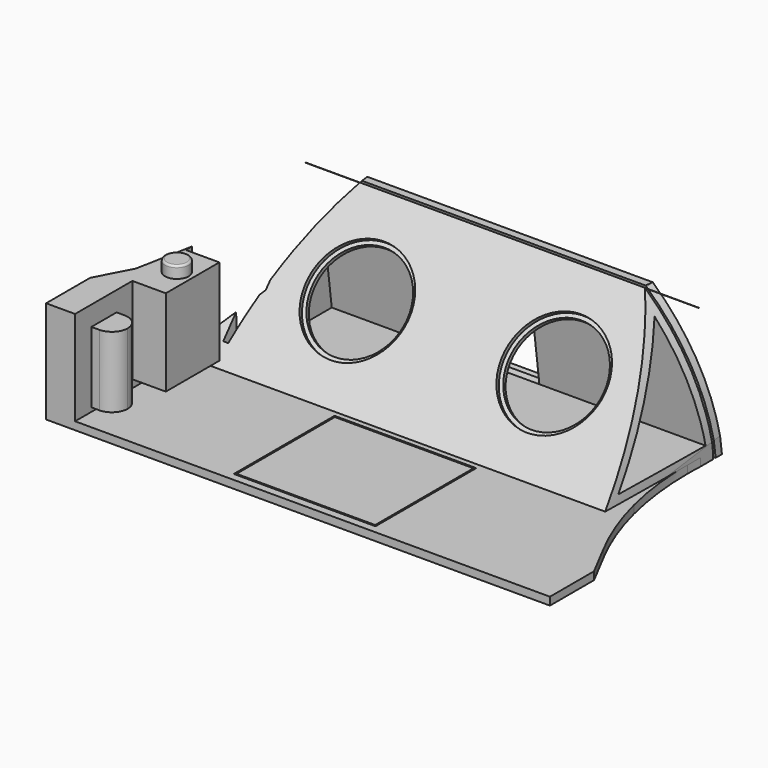
from build123d import *

# Parameters (mm, degrees)
F1_DEPTH  = 25.4
F3_DEPTH  = 1270
F5_W      = 457.2
F5_H      = 406.4
F6_DEPTH  = 25.4
F7_W      = 447.04
F7_H      = 396.24
F8_DEPTH  = 25.4
F10_DEPTH = 1358.9
F11_R     = 165.1
F12_DEPTH = 12.7
F14_DEPTH = 1206.5
F16_DEPTH = 25.4
F17_R     = 152.4
F18_DEPTH = 25.4
F4_W      = 203.2
F4_H      = 397.8725210062
F19_DEPTH = 25.4
F21_DEPTH = 25.4
F23_DEPTH = 459.74
F24_W     = 185.8009562355
F24_H     = 25.4
F25_DEPTH = 127
F27_DEPTH = 25.4
F29_DEPTH = 25.4
F31_DEPTH = 304.8
F32_W     = 215.9
F32_H     = 279.4
F33_DEPTH = 107.95
F34_W     = 101.6
F34_H     = 228.6
F35_DEPTH = 76.2
F36_R     = 50.8
F37_R     = 50.79999
F38_R     = 38.1
F39_DEPTH = 38.1
F40_R     = 6.35
F42_DEPTH = 508
F44_DEPTH = 406.4


# Not quite as in the source:
# - a fillet or chamfer is up to 0.001 mm smaller than in the source, because OpenCascade refuses the exact size


with BuildPart() as f1:
    # F0 (on Top) → F1 (new body)
    with BuildSketch(Plane.XY):
        Polygon((633.9916200739, 381), (-636.0083799261, 381), (-636.0083799261, 279.4), (-585.2083799261, 279.4), (-585.2083799261, 101.6), (-720.2711577423, -25.9932654437), (-755.401483878, -208.8168415053), (-813.8083799261, -320.4935488224), (-813.8083799261, -498.2935488224), (-636.0083799261, -498.2935488224), (633.9916200739, -498.2935488224), (811.7916200739, -498.2935488224), (811.7916200739, -320.4935488224), (753.3847240259, -208.8168415053), (718.2543978901, -25.9932654437), (583.1916200739, 101.6), (583.1916200739, 279.4), (633.9916200739, 279.4), align=None)
    extrude(amount=F1_DEPTH)

    # F5 (on face) → F6 (cut)
    with BuildSketch(Plane.XY.offset(25.4)):
        with Locations((0, -269.6935488224)):
            Rectangle(F5_W, F5_H)
    extrude(amount=-F6_DEPTH, mode=Mode.SUBTRACT)


with BuildPart() as f3:
    # F2 (on face) → F3 (new body)
    with BuildSketch(Plane.YZ.offset(633.9916200739)):
        Polygon((355.6, 457.2), (330.2, 457.2), (392.1093138361, 0), (417.5093138361, 0), align=None)
    extrude(amount=-F3_DEPTH)

    # F4 (on face) → F19 (cut)
    with BuildSketch(Plane(origin=(0, 385.0491351938, 52.1393870364), x_dir=(1, 0, 0), z_dir=(0, -0.9909562863, -0.1341850913))):
        with Locations((0, 184.4210364421)):
            Rectangle(F4_W, F4_H)
    extrude(amount=-F19_DEPTH, mode=Mode.SUBTRACT)

    # F20 (on face) → F21 (cut)
    with BuildSketch(Plane(origin=(0, 385.0491351938, 52.1393870364), x_dir=(1, 0, 0), z_dir=(0, -0.9909562863, -0.1341850913))):
        with BuildLine():
            ThreePointArc((-636.0083799261, -52.615224061), (-589.7862100298, 194.7614898935), (-457.3568999767, 408.7572969452))
            Line((-457.3568999767, 408.7572969452), (-636.0083799261, 408.7572969452))
            Line((-636.0083799261, 408.7572969452), (-636.0083799261, -52.615224061))
        make_face()
        with BuildLine():
            Line((633.9916200739, 408.7572969452), (457.3568999767, 408.7572969452))
            ThreePointArc((457.3568999767, 408.7572969452), (579.8251172789, 219.089488202), (633.9916200739, -0.0869975296))
            Line((633.9916200739, -0.0869975296), (633.9916200739, 408.7572969452))
        make_face()
    extrude(amount=-F21_DEPTH, mode=Mode.SUBTRACT)


with BuildPart() as f8:
    # F7 (on face) → F8 (new body)
    with BuildSketch(Plane.XY.offset(25.4)):
        with Locations((0, -269.6935488224)):
            Rectangle(F7_W, F7_H)
    extrude(amount=-F8_DEPTH)


with BuildPart() as f10:
    # F9 (on face) → F10 (new body)
    with BuildSketch(Plane.YZ.offset(633.9916200739)):
        Polygon((137.9962750452, 239.4747816958), (381, 25.4), (324.9715128924, 453.5495633916), align=None)
        Polygon((-48.9789628019, 25.4), (381, 25.4), (137.9962750452, 239.4747816958), align=None)
    extrude(amount=-F10_DEPTH)

    # F11 (on face) → F12 (cut)
    with BuildSketch(Plane(origin=(0, -40.3685730448, 35.2583498477), x_dir=(1, 0, 0), z_dir=(0, -0.7531695417, 0.6578264524))):
        with Locations((-318.5083799261, 271.1485742475)):
            Circle(F11_R)
        with Locations((316.4916200739, 271.1485742475)):
            Circle(F11_R)
    extrude(amount=-F12_DEPTH, mode=Mode.SUBTRACT)

    # F13 (on face) → F14 (cut)
    with BuildSketch(Plane.YZ.offset(633.9916200739)):
        Polygon((352.0595440659, 50.8), (307.0873524009, 394.4613269455), (6.9298194327, 50.8), align=None)
    extrude(amount=-F14_DEPTH, mode=Mode.SUBTRACT)

    # F15 (on face) → F16 (cut)
    with BuildSketch(Plane(origin=(0, 377.8532138761, 49.446608691), x_dir=(-1, 0, 0), z_dir=(0, 0.9915460014, 0.1297556441))):
        Polygon((105.7816183023, 356.7483680457), (-97.4728635717, 356.7483680457), (-97.4728635717, 1.383348692), (105.3700960746, 1.1486061652), align=None)
    extrude(amount=-F16_DEPTH, mode=Mode.SUBTRACT)

    # F17 (on face) → F18 (cut)
    with BuildSketch(Plane(origin=(0, -30.8033198656, 26.9039539021), x_dir=(1, 0, 0), z_dir=(0, -0.7531695417, 0.6578264524))):
        with Locations((-318.5083799261, 271.1485742475)):
            Circle(F17_R)
        with Locations((316.4916200739, 271.1485742475)):
            Circle(F17_R)
    extrude(amount=-F18_DEPTH, mode=Mode.SUBTRACT)


with BuildPart() as f23_tool:
    # F22 (on face) → F23 (new body)
    with BuildSketch(Plane(origin=(0, 409.9917919704, 55.5168646529), x_dir=(-1, 0, 0), z_dir=(0, 0.9909562863, 0.1341850913))):
        with BuildLine():
            ThreePointArc((-633.9916200739, -0.0869975295), (-580.1776273816, 216.7403618545), (-460.4411130957, 405.3489956272))
            Line((-460.4411130957, 405.3489956272), (-652.6208519936, 405.3489956272))
            Line((-652.6208519936, 405.3489956272), (-633.9916200739, -0.0869975295))
        make_face()
    extrude(amount=-F23_DEPTH)


with BuildPart() as f1_1:
    add(f1.part)

    # F23: cut by f23_tool
    add(f23_tool.part, mode=Mode.SUBTRACT)



with BuildPart() as f3_1:
    add(f3.part)

    # F23: cut by f23_tool
    add(f23_tool.part, mode=Mode.SUBTRACT)


with BuildPart() as f10_1:
    add(f10.part)

    # F23: cut by f23_tool
    add(f23_tool.part, mode=Mode.SUBTRACT)


with BuildPart() as f1_2:
    add(f1_1.part)

    add(f10_1.part)  # F25 merges F10
    # F24 (on face) → F25 (join)
    with BuildSketch(Plane(origin=(325.7420855468, 344.8115445011, 0), x_dir=(-0.726921866, 0.6867201764, 0), z_dir=(0.6867201764, 0.726921866, 0))):
        with Locations((-447.0644489093, 12.7)):
            Rectangle(F24_W, F24_H)
    extrude(amount=-F25_DEPTH)

    # F26 (on face) → F27 (join)
    with BuildSketch(Plane(origin=(0, 0, 0), x_dir=(1, 0, 0), z_dir=(0, 0, -1))):
        with BuildLine():
            ThreePointArc((633.9916200739, -330.2), (657.9193133131, -52.7687190683), (753.3847240259, 208.8168415053))
            Line((753.3847240259, 208.8168415053), (533.1680178642, 208.8168415053))
            Line((533.1680178642, 208.8168415053), (533.1680178642, -330.2))
            Line((533.1680178642, -330.2), (633.9916200739, -330.2))
        make_face()
    extrude(amount=-F27_DEPTH)

    # F28 (on face) → F29 (cut)
    with BuildSketch(Plane(origin=(0, 0, 0), x_dir=(1, 0, 0), z_dir=(0, 0, -1))):
        with BuildLine():
            Line((763.2642388344, -52.6611953974), (753.3847240259, 208.8168415053))
            ThreePointArc((753.3847240259, 208.8168415053), (657.9193133131, -52.7687190683), (633.9916200739, -330.2))
            Line((633.9916200739, -330.2), (763.2642388344, -52.6611953974))
        make_face()
    extrude(amount=-F29_DEPTH, mode=Mode.SUBTRACT)

    # F30 (on face) → F31 (join)
    with BuildSketch(Plane.XY.offset(25.4)):
        Polygon((-720.2711577423, -498.2935488224), (-720.2711577423, -25.9932654437), (-745.6711577423, -158.1787400112), (-755.401483878, -208.8168415053), (-813.8083799261, -320.4935488224), (-813.8083799261, -498.2935488224), (-745.6711577423, -498.2935488224), align=None)
    extrude(amount=F31_DEPTH)

    # F32 (on face) → F33 (join)
    with BuildSketch(Plane.YZ.offset(-720.2711577423)):
        with Locations((-159.3432654437, 190.5)):
            Rectangle(F32_W, F32_H)
    extrude(amount=F33_DEPTH)

    # F34 (on face) → F35 (join)
    with BuildSketch(Plane.YZ.offset(-720.2711577423)):
        with Locations((-381.5932654437, 152.4)):
            Rectangle(F34_W, F34_H)
    extrude(amount=F35_DEPTH)

    # F36
    f36_edges = [f1_2.edges().sort_by_distance(p)[0] for p in [
        (-644.071158, -432.393265, 152.4),
    ]]
    fillet(f36_edges, radius=F36_R)

    # F37 (radius 50.8 in the source; OpenCascade refuses exactly that, so slightly less here)
    f37_edges = [f1_2.edges().sort_by_distance(p)[0] for p in [
        (-644.071158, -330.793265, 152.4),
    ]]
    fillet(f37_edges, radius=F37_R)

    # F38 (on face) → F39 (join)
    with BuildSketch(Plane.XY.offset(330.2)):
        with Locations((-663.1211577423, -159.3432654437)):
            Circle(F38_R)
    extrude(amount=F39_DEPTH)

    # F40
    f40_edges = [f1_2.edges().sort_by_distance(p)[0] for p in [
        (-701.221158, -159.343265, 368.3),
    ]]
    fillet(f40_edges, radius=F40_R)

    # F41 (on face) → F42 (cut)
    with BuildSketch(Plane(origin=(0, 0, 0), x_dir=(1, 0, 0), z_dir=(0, 0, -1))):
        Polygon((-751.9905567169, -381), (-636.0083799261, -381), (-636.0083799261, -279.4), (-585.2083799261, -279.4), (-585.2083799261, -101.6), (-720.2711577423, 25.9932654437), (-724.7296735254, 49.1960616901), (-755.401483878, 78.8422897458), align=None)
    extrude(amount=-F42_DEPTH, mode=Mode.SUBTRACT)


with BuildPart() as f44_tool:
    # F43 (on face) → F44 (new body)
    with BuildSketch(Plane(origin=(0, 409.9917919704, 55.5168646529), x_dir=(-1, 0, 0), z_dir=(0, 0.9909562863, 0.1341850913))):
        with BuildLine():
            ThreePointArc((460.4411130957, 405.3489956272), (586.8395822523, 197.335702788), (635.9111193057, -41.0716948618))
            Line((635.9111193057, -41.0716948618), (645.3213691711, 405.3489956272))
            Line((645.3213691711, 405.3489956272), (460.4411130957, 405.3489956272))
        make_face()
    extrude(amount=-F44_DEPTH)


with BuildPart() as f1_3:
    add(f1_2.part)

    # F44: cut by f44_tool
    add(f44_tool.part, mode=Mode.SUBTRACT)


with BuildPart() as f3_2:
    add(f3_1.part)

    # F44: cut by f44_tool
    add(f44_tool.part, mode=Mode.SUBTRACT)


solid = Compound([f8.part, f1_3.part, f3_2.part])
